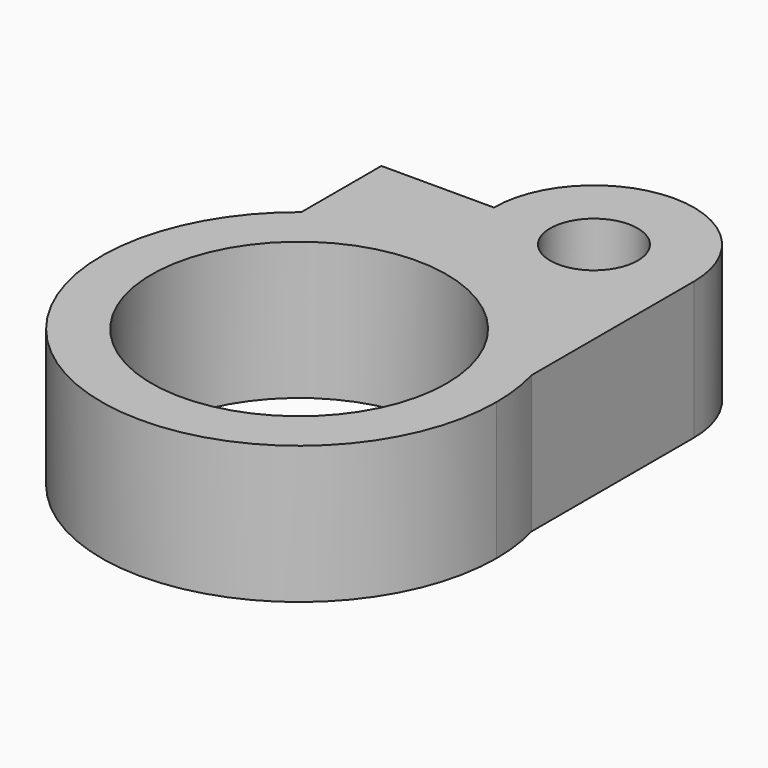
from build123d import *

# Parameters (mm, degrees)
F0_R     = 1.75
F0_R_2   = 5.9
F1_DEPTH = 5.5
F2_R     = 3.99999


# Not quite as in the source:
# - a fillet or chamfer is up to 0.001 mm smaller than in the source, because OpenCascade refuses the exact size


with BuildPart() as f1:
    # F0 (on Top) → F1 (new body)
    with BuildSketch(Plane.XY):
        with BuildLine():
            ThreePointArc((-4.881075218, 6.2116909708), (2.4746829154, 7.5023959152), (7.618924782, 2.0885366088))
            Line((7.618924782, 2.0885366088), (7.618924782, 14.2116909708))
            Line((7.618924782, 14.2116909708), (-0.381075218, 14.2116909708))
            Line((-0.381075218, 14.2116909708), (-0.381075218, 10.2116909708))
            Line((-0.381075218, 10.2116909708), (-4.881075218, 10.2116909708))
            Line((-4.881075218, 10.2116909708), (-4.881075218, 6.2116909708))
        make_face()
        with Locations((3.618924782, 10.2116909708)):
            Circle(F0_R, mode=Mode.SUBTRACT)
        with BuildLine():
            ThreePointArc((-4.881075218, 6.2116909708), (-3.4532235504, -7.1052971163), (7.9, 0))
            ThreePointArc((7.9, 0), (7.8294158715, 1.0536826425), (7.618924782, 2.0885366088))
            ThreePointArc((7.618924782, 2.0885366088), (2.4746829154, 7.5023959152), (-4.881075218, 6.2116909708))
        make_face()
        Circle(F0_R_2, mode=Mode.SUBTRACT)
    extrude(amount=F1_DEPTH)

    # F2 (radius 4 in the source; OpenCascade refuses exactly that, so slightly less here)
    f2_edges = [f1.edges().sort_by_distance(p)[0] for p in [
        (-0.381075, 14.211691, 2.75),
        (7.618925, 14.211691, 2.75),
    ]]
    fillet(f2_edges, radius=F2_R)


solid = f1.part
